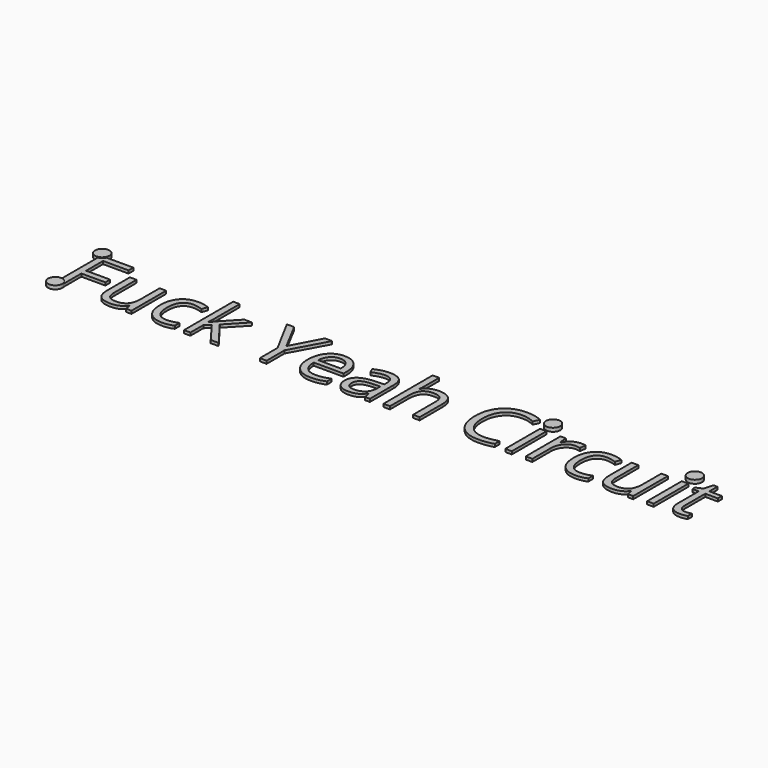
from build123d import *

# Parameters (mm, degrees)
F0_TEXT_SIZE = 11.2876991515
F1_DEPTH     = 0.4
F2_R         = 1
F3_DEPTH     = 0.5


# Not quite as in the source:
# - Text() gives the source's letters only with a copy of the font that has no kerning and outlines rounded to 1/6400 em; it was checked with that copy


with BuildPart() as f1:
    # F0 (on Top) → F1 (new body)
    with BuildSketch(Plane.XY):
        with Locations((-10.2209162982, -2.0386733696)):
            Text('Fuck Yeah Circuit', F0_TEXT_SIZE, font='Open Sans', text_align=(TextAlign.LEFT, TextAlign.BOTTOM))
    extrude(amount=F1_DEPTH)


with BuildPart() as f3:
    # F2 (on Top) → F3 (new body)
    with BuildSketch(Plane.XY):
        with Locations((-9.289235808, 6.4350427128)):
            Circle(F2_R)
    extrude(amount=F3_DEPTH)


with BuildPart() as f3b:
    # F2 (on Top) → F3, piece 2 (new body)
    with BuildSketch(Plane.XY):
        with Locations((-9.1398153454, -1.9325403264)):
            Circle(F2_R)
    extrude(amount=F3_DEPTH)


with BuildPart() as f3c:
    # F2 (on Top) → F3, piece 3 (new body)
    with BuildSketch(Plane.XY):
        with Locations((54.1123859584, 5.7043912821)):
            Circle(F2_R)
    extrude(amount=F3_DEPTH)


with BuildPart() as f3d:
    # F2 (on Top) → F3, piece 4 (new body)
    with BuildSketch(Plane.XY):
        with Locations((73.8111436367, 5.7752272114)):
            Circle(F2_R)
    extrude(amount=F3_DEPTH)


solid = Compound([f1.part, f3.part, f3b.part, f3c.part, f3d.part])
